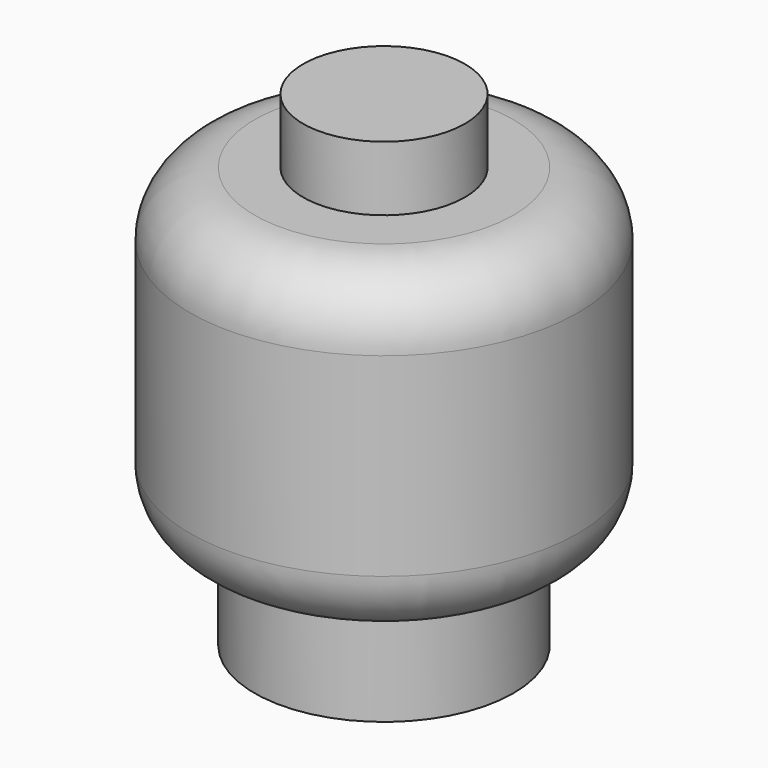
from build123d import *

# Parameters (mm, degrees)
F0_R     = 4
F1_DEPTH = 3
F2_R     = 6
F3_DEPTH = 10
F4_R     = 2.5
F5_DEPTH = 2
F6_R     = 1.99999
F7_R     = 2.5
F8_DEPTH = 8


# Not quite as in the source:
# - a fillet or chamfer is up to 0.001 mm smaller than in the source, because OpenCascade refuses the exact size
# - a feature names something its author has since deleted; it is built from what else it names


with BuildPart() as f1:
    # F0 (on Top) → F1 (new body)
    with BuildSketch(Plane.XY):
        Circle(F0_R)
    extrude(amount=F1_DEPTH)

    # F2 (on face) → F3 (join)
    with BuildSketch(Plane.XY.offset(3)):
        Circle(F2_R)
    extrude(amount=F3_DEPTH)

    # F4 (on face) → F5 (join)
    with BuildSketch(Plane.XY.offset(13)):
        Circle(F4_R)
    extrude(amount=F5_DEPTH)

    # F6 (radius 2 in the source; OpenCascade refuses exactly that, so slightly less here)
    f6_edges = [f1.edges().sort_by_distance(p)[0] for p in [
        (-6, 0, 13),
        (-6, 0, 3),
    ]]
    fillet(f6_edges, radius=F6_R)

    # F7 (on face) → F8 (cut)
    with BuildSketch(Plane(origin=(0, 0, 0), x_dir=(1, 0, 0), z_dir=(0, 0, -1))):
        Circle(F7_R)
    extrude(amount=-F8_DEPTH, mode=Mode.SUBTRACT)


solid = f1.part
